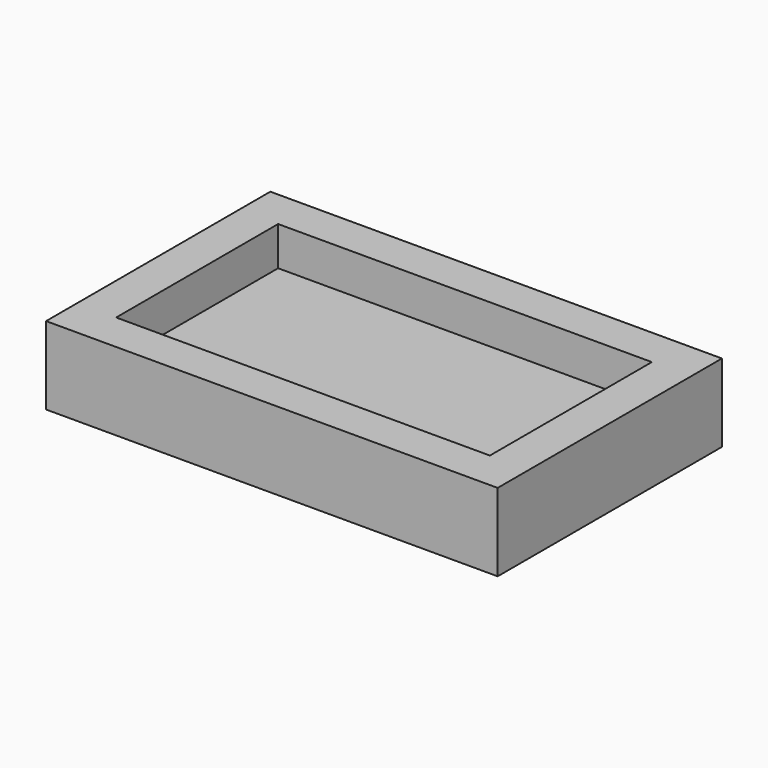
from build123d import *

# Parameters (mm, degrees)
F0_W     = 58
F0_H     = 36
F0_W_2   = 48
F0_H_2   = 26
F1_DEPTH = 5
F2_DEPTH = 10
F3_W     = 15
F3_H     = 5
F4_DEPTH = 15
F5_R     = 2.5
F6_DEPTH = 25
F7_R     = 5


# Not quite as in the source:
# - a feature names something its author has since deleted; it is built from what else it names


with BuildPart() as f1:
    # F0 (on Top) → F1 (new body)
    with BuildSketch(Plane.XY):
        with Locations((1.3224579843, 19.3690634753)):
            Rectangle(F0_W, F0_H)
        with Locations((1.3224579843, 19.3690634753)):
            Rectangle(F0_W_2, F0_H_2, mode=Mode.SUBTRACT)
        with Locations((1.3224579843, 19.3690634753)):
            Rectangle(F0_W_2, F0_H_2)
    extrude(amount=F1_DEPTH)

    # F0 (on Top) → F2 (join)
    with BuildSketch(Plane.XY):
        with Locations((1.3224579843, 19.3690634753)):
            Rectangle(F0_W, F0_H)
        with Locations((1.3224579843, 19.3690634753)):
            Rectangle(F0_W_2, F0_H_2, mode=Mode.SUBTRACT)
    extrude(amount=F2_DEPTH)

    # F3 (on face) → F4 (join)
    with BuildSketch(Plane(origin=(0, 0, 0), x_dir=(1, 0, 0), z_dir=(0, 0, -1))):
        with Locations((1.3224579843, -34.8690634753)):
            Rectangle(F3_W, F3_H)
    extrude(amount=F4_DEPTH)

    # F5 (on face) → F6 (cut)
    with BuildSketch(Plane.XZ.offset(-32.3690634753)):
        with Locations((1.3224579843, -7.5)):
            Circle(F5_R)
    extrude(amount=-F6_DEPTH, mode=Mode.SUBTRACT)

    # F7
    f7_edges = [f1.edges().sort_by_distance(p)[0] for p in [
        (8.822458, 34.869063, -15),
        (-6.177542, 34.869063, -15),
        (8.822458, 34.869063, 0),
        (-6.177542, 34.869063, 0),
    ]]
    fillet(f7_edges, radius=F7_R)


solid = f1.part
